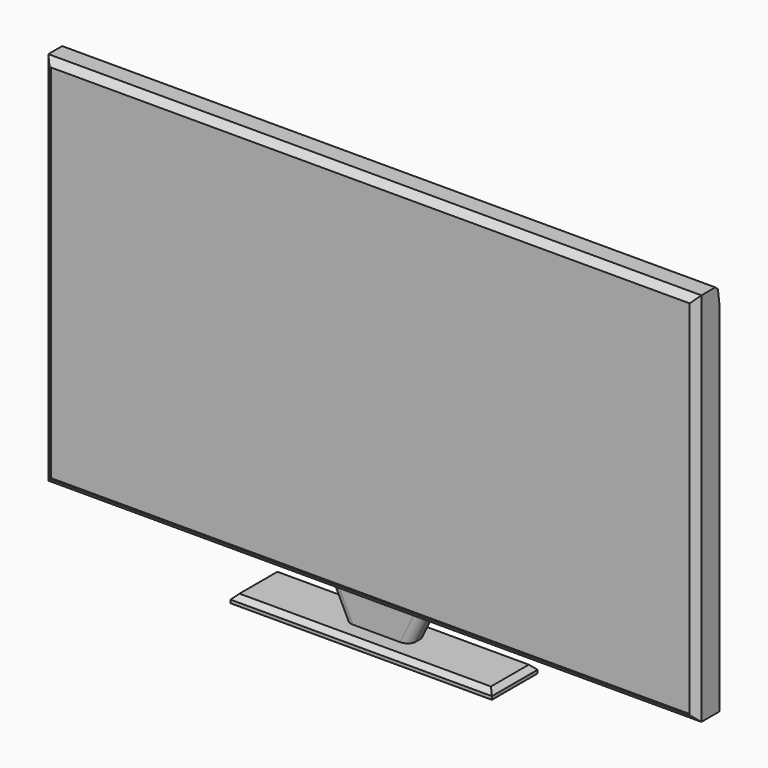
from build123d import *

# Parameters (mm, degrees)
F1_DEPTH     = 5.08
F3_DEPTH     = 0.508
F4_SIZE      = 1.016
F5_SIZE      = 1.016
F6_SIZE      = 1.016
F7_SIZE      = 1.016
F9_DEPTH     = 101.6
F10_DEPTH    = 4.7498
F11_DEPTH    = 1.397
F13_DEPTH    = 1.27
F14_R        = 1.27
F15_SIZE     = 0.762
F16_T1_DEPTH = 56.929231961
F16_T3_DEPTH = 104.2128299158
F16_T5_DEPTH = 103.8931341765
F17_DEPTH    = 0.254
F18_DEPTH    = 0.0254
F19_W        = 0.3161691129
F19_H        = 5.5101290345
F20_DEPTH    = 0.254
F21_W        = 1.812425442
F21_H        = 13.0091449246
F22_DEPTH    = 0.254
F23_R        = 0.5959561868
F24_DEPTH    = 0.381
F25_R        = 0.254
F26_W        = 7.7789444476
F26_H        = 3.8154134527
F27_DEPTH    = 1.27
F28_DEPTH    = 0.0254
F29_R        = 0.9198153673
F30_R        = 0.6978572148
F30_R_2      = 0.4079357796
F31_DEPTH    = 0.762


# Not quite as in the source:
# - a fillet or chamfer that OpenCascade refuses, or shapes differently, is made with other operations: its cross-section is extruded or revolved along the edge and cut away or added


with BuildPart() as f1:
    # F0 (on Front) → F1 (new body)
    with BuildSketch(Plane.XZ):
        Polygon((54.1567845821, 48.2408194919), (-47.4432154179, 48.2408194919), (-47.4432154179, -10.1791805081), (-3.9702162342, -10.1791805081), (10.6325710388, -10.1791805081), (54.1567845821, -10.1791805081), align=None)
    extrude(amount=-F1_DEPTH)

    # F2 (on face) → F3 (cut)
    with BuildSketch(Plane.XZ):
        Polygon((52.1729253232, 49.4569726288), (-45.6269144039, 49.4569726288), (-45.6223424486, 48.2408194919), (52.1729253232, 48.2408194919), align=None)
    extrude(amount=-F3_DEPTH, mode=Mode.SUBTRACT)

    # F4
    f4_edges = [f1.edges().sort_by_distance(p)[0] for p in [
        (-47.443215, 0, 19.030819),
    ]]
    chamfer(f4_edges, length=F4_SIZE)

    # F5
    f5_edges = [f1.edges().sort_by_distance(p)[0] for p in [
        (3.864785, 0, 48.240819),
    ]]
    chamfer(f5_edges, length=F5_SIZE)

    # F6
    f6_edges = [f1.edges().sort_by_distance(p)[0] for p in [
        (54.156785, 0, 18.522819),
    ]]
    chamfer(f6_edges, length=F6_SIZE)

    # F7
    f7_edges = [f1.edges().sort_by_distance(p)[0] for p in [
        (3.356785, 0, -10.179181),
    ]]
    chamfer(f7_edges, length=F7_SIZE)

    # F8 (on face) → F9 (cut, through all)
    with BuildSketch(Plane.YZ.offset(54.1567845821)):
        Polygon((5.08, 48.2408194919), (4.159392789, 48.2408194919), (5.08, 41.5243916214), align=None)
    extrude(amount=-F9_DEPTH, mode=Mode.SUBTRACT)

    # F16: chamfer of 0.508 on 4 edges, made by hand

    # F16_s2 → F16_t1 (cut)
    with BuildSketch(Plane.XY.offset(-11.485595466)):
        Polygon((-47.4432154179, 4.572), (-46.9352154179, 5.08), (-47.4432154179, 5.08), align=None)
        Polygon((54.1567845821, 4.572), (53.6487845821, 5.08), (54.1567845821, 5.08), align=None)
    extrude(amount=F16_T1_DEPTH, mode=Mode.SUBTRACT)

    # F16_s4 → F16_t3 (cut)
    with BuildSketch(Plane.YZ.offset(-48.7496303757)):
        Polygon((4.572, -10.1791805081), (5.08, -9.6711805081), (5.08, -10.1791805081), align=None)
    extrude(amount=F16_T3_DEPTH, mode=Mode.SUBTRACT)

    # F16_s6 → F16_t5 (cut)
    with BuildSketch(Plane.YZ.offset(-48.5897825061)):
        Polygon((3.716273471, 48.2408194919), (4.2195676186, 47.8018050048), (4.159392789, 48.2408194919), align=None)
    extrude(amount=F16_T5_DEPTH, mode=Mode.SUBTRACT)

    # F17 (cut): a face of the model
    f17_faces = [f1.faces().sort_by_distance(p)[0] for p in [
        (3.3567845821, 0, 19.0308194919),
    ]]
    extrude(f17_faces, amount=-F17_DEPTH, mode=Mode.SUBTRACT)


with BuildPart() as f10:
    # F0 (on Front) → F10 (new body)
    with BuildSketch(Plane.XZ):
        Polygon((10.6325710388, -10.1791805081), (-3.9702162342, -10.1791805081), (-1.7488225977, -14.7477481514), (3.3311774023, -14.7477481514), (8.4111774023, -14.7477481514), align=None)
    extrude(amount=-F10_DEPTH)

    # F11 (cut): a face of the model
    f11_faces = [f10.faces().sort_by_distance(p)[0] for p in [
        (3.3311774023, 0, -12.3268536031),
    ]]
    extrude(f11_faces, amount=-F11_DEPTH, mode=Mode.SUBTRACT)

    # F12 (on face) → F13 (join)
    with BuildSketch(Plane(origin=(0, 0, -14.7477481514), x_dir=(1, 0, 0), z_dir=(0, 0, -1))):
        Polygon((3.3311774023, -4.7498), (3.3311774023, -3.0734), (3.3311774023, -1.397), (-1.7488225977, -1.397), (-1.7488225977, -4.7498), align=None)
        Polygon((3.3311774023, -1.397), (3.3311774023, -3.0734), (3.3311774023, -4.7498), (8.4111774023, -4.7498), (8.4111774023, -1.397), align=None)
        Polygon((-1.7488225977, -1.397), (3.3311774023, -1.397), (3.3311774023, 1.590716306), (-16.9888225977, 1.590716306), (-16.9888225977, -7.299283694), (3.3311774023, -7.299283694), (3.3311774023, -4.7498), (-1.7488225977, -4.7498), align=None)
        Polygon((3.3311774023, 1.590716306), (3.3311774023, -1.397), (8.4111774023, -1.397), (8.4111774023, -4.7498), (3.3311774023, -4.7498), (3.3311774023, -7.299283694), (23.6511774023, -7.299283694), (23.6511774023, 1.590716306), align=None)
    extrude(amount=F13_DEPTH)

    # F14
    f14_edges = [f10.edges().sort_by_distance(p)[0] for p in [
        (-2.859519, 4.7498, -12.463464),
        (-2.859519, 1.397, -12.463464),
        (9.521874, 1.397, -12.463464),
        (9.521874, 4.7498, -12.463464),
    ]]
    fillet(f14_edges, radius=F14_R)

    # F15
    f15_edges = [f10.edges().sort_by_distance(p)[0] for p in [
        (-16.988823, 2.854284, -14.747748),
        (3.331177, -1.590716, -14.747748),
        (23.651177, 2.854284, -14.747748),
        (3.331177, 7.299284, -14.747748),
    ]]
    chamfer(f15_edges, length=F15_SIZE)


with BuildPart() as f18:
    # F18 (new): a face of the model
    f18_faces = [f1.part.faces().sort_by_distance(p)[0] for p in [
        (3.3567845821, 0.254, 19.0308194919),
    ]]
    extrude(f18_faces, amount=F18_DEPTH)


with BuildPart() as f1_1:
    add(f1.part)

    # F19 (on face) → F20 (cut)
    with BuildSketch(Plane(origin=(0, 10.5730224909, 1.449222851), x_dir=(-1, 0, 0), z_dir=(0, 0.990736511, 0.1357982537))):
        with Locations((-53.1502272934, 43.5757227242)):
            Rectangle(F19_W, F19_H)
        with Locations((-51.1182272934, 43.5757227242)):
            Rectangle(F19_W, F19_H)
        with Locations((-49.0862272934, 43.5757227242)):
            Rectangle(F19_W, F19_H)
        with Locations((-47.0542272934, 43.5757227242)):
            Rectangle(F19_W, F19_H)
        with Locations((-45.0222272934, 43.5757227242)):
            Rectangle(F19_W, F19_H)
        with Locations((-42.9902272934, 43.5757227242)):
            Rectangle(F19_W, F19_H)
        with Locations((-40.9582272934, 43.5757227242)):
            Rectangle(F19_W, F19_H)
        with Locations((-38.9262272934, 43.5757227242)):
            Rectangle(F19_W, F19_H)
        with Locations((-36.8942272934, 43.5757227242)):
            Rectangle(F19_W, F19_H)
        with Locations((-34.8622272934, 43.5757227242)):
            Rectangle(F19_W, F19_H)
        with Locations((-32.8302272934, 43.5757227242)):
            Rectangle(F19_W, F19_H)
        with Locations((-30.7982272934, 43.5757227242)):
            Rectangle(F19_W, F19_H)
        with Locations((-28.7662272934, 43.5757227242)):
            Rectangle(F19_W, F19_H)
        with Locations((-26.7342272934, 43.5757227242)):
            Rectangle(F19_W, F19_H)
        with Locations((-24.7022272934, 43.5757227242)):
            Rectangle(F19_W, F19_H)
        with Locations((-22.6702272934, 43.5757227242)):
            Rectangle(F19_W, F19_H)
        with Locations((-20.6382272934, 43.5757227242)):
            Rectangle(F19_W, F19_H)
        with Locations((-18.6062272934, 43.5757227242)):
            Rectangle(F19_W, F19_H)
        with Locations((-16.5742272934, 43.5757227242)):
            Rectangle(F19_W, F19_H)
        with Locations((-14.5422272934, 43.5757227242)):
            Rectangle(F19_W, F19_H)
        with Locations((-12.5102272934, 43.5757227242)):
            Rectangle(F19_W, F19_H)
        with Locations((-10.4782272934, 43.5757227242)):
            Rectangle(F19_W, F19_H)
        with Locations((-8.4462272934, 43.5757227242)):
            Rectangle(F19_W, F19_H)
        with Locations((-6.4142272934, 43.5757227242)):
            Rectangle(F19_W, F19_H)
        with Locations((-4.3822272934, 43.5757227242)):
            Rectangle(F19_W, F19_H)
        with Locations((-2.3502272934, 43.5757227242)):
            Rectangle(F19_W, F19_H)
        with Locations((-0.3182272934, 43.5757227242)):
            Rectangle(F19_W, F19_H)
        with Locations((1.7137727066, 43.5757227242)):
            Rectangle(F19_W, F19_H)
        with Locations((3.7457727066, 43.5757227242)):
            Rectangle(F19_W, F19_H)
        with Locations((5.7777727066, 43.5757227242)):
            Rectangle(F19_W, F19_H)
        with Locations((7.8097727066, 43.5757227242)):
            Rectangle(F19_W, F19_H)
        with Locations((9.8417727066, 43.5757227242)):
            Rectangle(F19_W, F19_H)
        with Locations((11.8737727066, 43.5757227242)):
            Rectangle(F19_W, F19_H)
        with Locations((13.9057727066, 43.5757227242)):
            Rectangle(F19_W, F19_H)
        with Locations((15.9377727066, 43.5757227242)):
            Rectangle(F19_W, F19_H)
        with Locations((17.9697727066, 43.5757227242)):
            Rectangle(F19_W, F19_H)
        with Locations((20.0017727066, 43.5757227242)):
            Rectangle(F19_W, F19_H)
        with Locations((22.0337727066, 43.5757227242)):
            Rectangle(F19_W, F19_H)
        with Locations((24.0657727066, 43.5757227242)):
            Rectangle(F19_W, F19_H)
        with Locations((26.0977727066, 43.5757227242)):
            Rectangle(F19_W, F19_H)
        with Locations((28.1297727066, 43.5757227242)):
            Rectangle(F19_W, F19_H)
        with Locations((30.1617727066, 43.5757227242)):
            Rectangle(F19_W, F19_H)
        with Locations((32.1937727066, 43.5757227242)):
            Rectangle(F19_W, F19_H)
        with Locations((34.2257727066, 43.5757227242)):
            Rectangle(F19_W, F19_H)
        with Locations((36.2577727066, 43.5757227242)):
            Rectangle(F19_W, F19_H)
        with Locations((38.2897727066, 43.5757227242)):
            Rectangle(F19_W, F19_H)
        with Locations((40.3217727066, 43.5757227242)):
            Rectangle(F19_W, F19_H)
        with Locations((42.3537727066, 43.5757227242)):
            Rectangle(F19_W, F19_H)
        with Locations((44.3857727066, 43.5757227242)):
            Rectangle(F19_W, F19_H)
        with Locations((46.4177727066, 43.5757227242)):
            Rectangle(F19_W, F19_H)
    extrude(amount=-F20_DEPTH, mode=Mode.SUBTRACT)

    # F21 (on face) → F22 (cut)
    with BuildSketch(Plane(origin=(-47.4432154179, 0, 0), x_dir=(0, -1, 0), z_dir=(-1, 0, 0))):
        with Locations((-2.786017023, -2.4052080698)):
            Rectangle(F21_W, F21_H)
    extrude(amount=-F22_DEPTH, mode=Mode.SUBTRACT)

    # F25
    f25_edges = [f1_1.edges().sort_by_distance(p)[0] for p in [
        (-47.316215, 3.69223, 4.099364),
        (-47.316215, 1.879804, 4.099364),
        (-47.316215, 1.879804, -8.909781),
        (-47.316215, 3.69223, -8.909781),
    ]]
    fillet(f25_edges, radius=F25_R)

    # F26 (on face) → F27 (cut)
    with BuildSketch(Plane(origin=(0, 5.08, 0), x_dir=(-1, 0, 0), z_dir=(0, 1, 0))):
        with Locations((17.0829044655, 11.9089582004)):
            Rectangle(F26_W, F26_H)
    extrude(amount=-F27_DEPTH, mode=Mode.SUBTRACT)


with BuildPart() as f24:
    # F23 (on face) → F24 (new body)
    with BuildSketch(Plane(origin=(-47.1892154179, 0, 0), x_dir=(0, -1, 0), z_dir=(-1, 0, 0))):
        with Locations((-2.786017023, -7.3206862435)):
            Circle(F23_R)
    extrude(amount=F24_DEPTH)


with BuildPart() as f24b:
    # F23 (on face) → F24, piece 2 (new body)
    with BuildSketch(Plane(origin=(-47.1892154179, 0, 0), x_dir=(0, -1, 0), z_dir=(-1, 0, 0))):
        with Locations((-2.7832970291, -5.669688484)):
            Circle(F23_R)
    extrude(amount=F24_DEPTH)


with BuildPart() as f24c:
    # F23 (on face) → F24, piece 3 (new body)
    with BuildSketch(Plane(origin=(-47.1892154179, 0, 0), x_dir=(0, -1, 0), z_dir=(-1, 0, 0))):
        with Locations((-2.7805770352, -4.0186907246)):
            Circle(F23_R)
    extrude(amount=F24_DEPTH)


with BuildPart() as f24d:
    # F23 (on face) → F24, piece 4 (new body)
    with BuildSketch(Plane(origin=(-47.1892154179, 0, 0), x_dir=(0, -1, 0), z_dir=(-1, 0, 0))):
        with Locations((-2.7778570414, -2.3676929652)):
            Circle(F23_R)
    extrude(amount=F24_DEPTH)


with BuildPart() as f24e:
    # F23 (on face) → F24, piece 5 (new body)
    with BuildSketch(Plane(origin=(-47.1892154179, 0, 0), x_dir=(0, -1, 0), z_dir=(-1, 0, 0))):
        with Locations((-2.7751370475, -0.7166952058)):
            Circle(F23_R)
    extrude(amount=F24_DEPTH)


with BuildPart() as f24f:
    # F23 (on face) → F24, piece 6 (new body)
    with BuildSketch(Plane(origin=(-47.1892154179, 0, 0), x_dir=(0, -1, 0), z_dir=(-1, 0, 0))):
        with Locations((-2.7724170536, 0.9343025537)):
            Circle(F23_R)
    extrude(amount=F24_DEPTH)


with BuildPart() as f24g:
    # F23 (on face) → F24, piece 7 (new body)
    with BuildSketch(Plane(origin=(-47.1892154179, 0, 0), x_dir=(0, -1, 0), z_dir=(-1, 0, 0))):
        with Locations((-2.7696970597, 2.5853003131)):
            Circle(F23_R)
    extrude(amount=F24_DEPTH)


with BuildPart() as f28:
    # F28 (new): a face of the model
    f28_faces = [f1_1.part.faces().sort_by_distance(p)[0] for p in [
        (-17.0829044655, 3.81, 11.9089582004),
    ]]
    extrude(f28_faces, amount=F28_DEPTH)


with BuildPart() as f1_2:
    add(f1_1.part)

    # F29
    f29_edges = [f1_2.edges().sort_by_distance(p)[0] for p in [
        (-13.193432, 4.445, 13.816665),
        (-13.193432, 4.445, 10.001251),
        (-20.972377, 4.445, 10.001251),
        (-20.972377, 4.445, 13.816665),
    ]]
    fillet(f29_edges, radius=F29_R)


with BuildPart() as f31:
    # F30 (on face) → F31 (new body)
    with BuildSketch(Plane(origin=(0, 3.8354, 0), x_dir=(-1, 0, 0), z_dir=(0, 1, 0))):
        with Locations((15.0926439092, 11.8966288865)):
            Circle(F30_R)
        with Locations((15.0926439092, 11.8966288865)):
            Circle(F30_R_2, mode=Mode.SUBTRACT)
    extrude(amount=F31_DEPTH)


with BuildPart() as f31b:
    # F30 (on face) → F31, piece 2 (new body)
    with BuildSketch(Plane(origin=(0, 3.8354, 0), x_dir=(-1, 0, 0), z_dir=(0, 1, 0))):
        with Locations((16.9722439092, 11.8966288865)):
            Circle(F30_R)
        with Locations((16.9722439092, 11.8966288865)):
            Circle(F30_R_2, mode=Mode.SUBTRACT)
    extrude(amount=F31_DEPTH)


with BuildPart() as f31c:
    # F30 (on face) → F31, piece 3 (new body)
    with BuildSketch(Plane(origin=(0, 3.8354, 0), x_dir=(-1, 0, 0), z_dir=(0, 1, 0))):
        with Locations((18.8518439092, 11.8966288865)):
            Circle(F30_R)
        with Locations((18.8518439092, 11.8966288865)):
            Circle(F30_R_2, mode=Mode.SUBTRACT)
    extrude(amount=F31_DEPTH)


solid = Compound([f10.part, f18.part, f24.part, f24b.part, f24c.part, f24d.part, f24e.part, f24f.part, f24g.part, f28.part, f1_2.part, f31.part, f31b.part, f31c.part])
